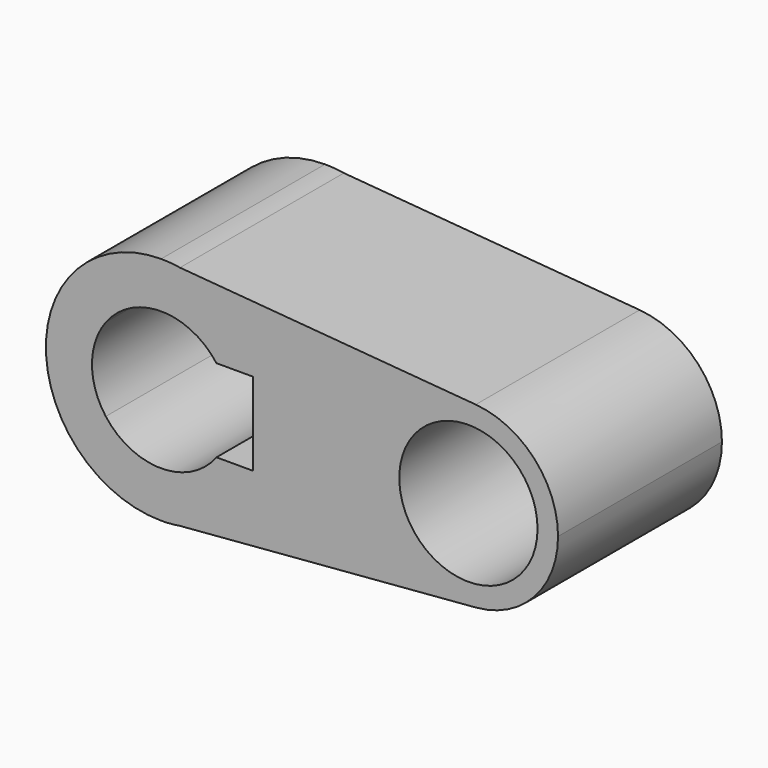
from build123d import *

# Parameters (mm, degrees)
F0_R     = 17.145
F1_DEPTH = 50.8


# Not quite as in the source:
# - a feature names something its author has since deleted; it is built from what else it names


with BuildPart() as f1:
    # F0 (on Front) → F1 (new body)
    with BuildSketch(Plane.XZ):
        with BuildLine():
            Line((4.6743845872, 28.1900825421), (0, 28.575))
            ThreePointArc((0, 28.575), (-28.575, 0), (0, -28.575))
            Line((0, -28.575), (4.6743845872, -28.1900825421))
            ThreePointArc((4.6743845872, -28.1900825421), (21.7956551241, -18.4791786265), (28.575, 0))
            ThreePointArc((28.575, 0), (21.7956551241, 18.4791786265), (4.6743845872, 28.1900825421))
        make_face()
        with BuildLine():
            ThreePointArc((-13.7262649311, -10.27329918), (-17.145, 0), (-13.7262649311, 10.27329918))
            ThreePointArc((-13.7262649311, 10.27329918), (0, 17.145), (13.7262649311, 10.27329918))
            Line((13.7262649311, 10.27329918), (22.7799285203, 10.27329918))
            Line((22.7799285203, 10.27329918), (22.7799285203, -10.27329918))
            Line((22.7799285203, -10.27329918), (13.7262649311, -10.27329918))
            ThreePointArc((13.7262649311, -10.27329918), (0, -17.145), (-13.7262649311, -10.27329918))
        make_face(mode=Mode.SUBTRACT)
        with BuildLine():
            ThreePointArc((4.6743845872, 28.1900825421), (2.3451030211, 28.4786080562), (0, 28.575))
            Line((0, 28.575), (4.6743845872, 28.1900825421))
        make_face()
        with BuildLine():
            Line((4.6743845872, -28.1900825421), (0, -28.575))
            ThreePointArc((0, -28.575), (2.3451030211, -28.4786080562), (4.6743845872, -28.1900825421))
        make_face()
        with BuildLine():
            Line((78.0239690164, 22.1500284882), (4.6743845872, 28.1900825421))
            ThreePointArc((4.6743845872, 28.1900825421), (21.7956551241, 18.4791786265), (28.575, 0))
            ThreePointArc((28.575, 0), (21.7956551241, -18.4791786265), (4.6743845872, -28.1900825421))
            Line((4.6743845872, -28.1900825421), (78.0239690164, -22.1500284882))
            ThreePointArc((78.0239690164, -22.1500284882), (53.975, 0), (78.0239690164, 22.1500284882))
        make_face()
        with BuildLine():
            ThreePointArc((98.425, 0), (92.5476043564, 15.0567744489), (78.0239690164, 22.1500284882))
            ThreePointArc((78.0239690164, 22.1500284882), (53.975, 0), (78.0239690164, -22.1500284882))
            ThreePointArc((78.0239690164, -22.1500284882), (92.5476043564, -15.0567744489), (98.425, 0))
        make_face()
        with Locations((76.2, 0)):
            Circle(F0_R, mode=Mode.SUBTRACT)
    extrude(amount=F1_DEPTH)


solid = f1.part
